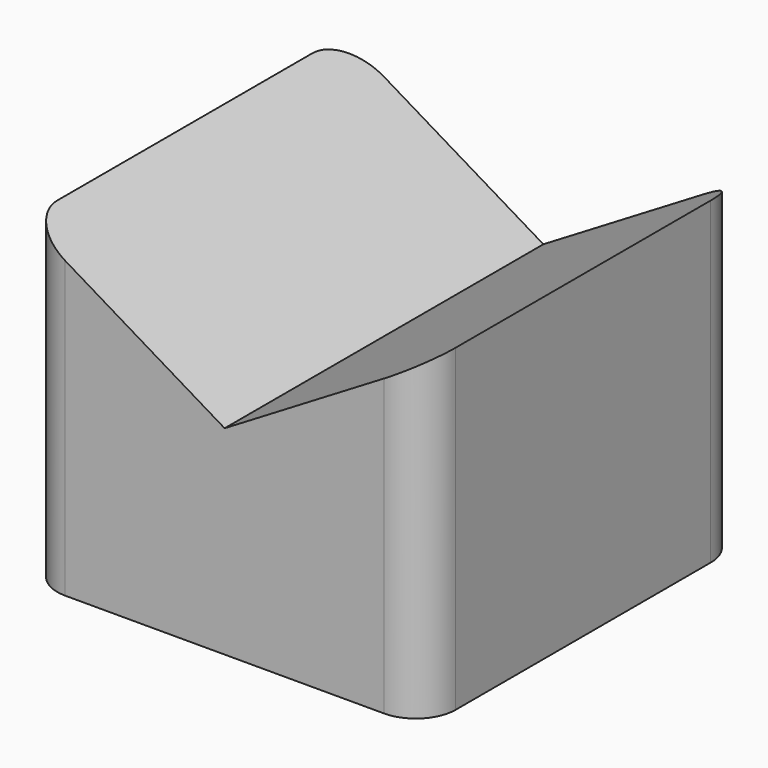
from build123d import *

# Parameters (mm, degrees)
F1_DEPTH = 20.32
F4_DEPTH = 25.4


with BuildPart() as f1:
    # F0 (on Top) → F1 (new body)
    with BuildSketch(Plane.XY):
        with BuildLine():
            Line((22.86, 0), (2.54, 0))
            ThreePointArc((2.54, 0), (0.7439487758, -0.7439487758), (0, -2.54))
            Line((0, -2.54), (0, -22.86))
            ThreePointArc((0, -22.86), (0.7439487758, -24.6560512242), (2.54, -25.4))
            Line((2.54, -25.4), (22.86, -25.4))
            ThreePointArc((22.86, -25.4), (24.6560512242, -24.6560512242), (25.4, -22.86))
            Line((25.4, -22.86), (25.4, -2.54))
            ThreePointArc((25.4, -2.54), (24.6560512242, -0.7439487758), (22.86, 0))
        make_face()
    extrude(amount=F1_DEPTH)

    # F2 (on face) → F4 (cut)
    with BuildSketch(Plane.XZ.offset(25.4)):
        Polygon((2.54, 18.796), (12.7, 12.7), (22.86, 18.796), (22.86, 20.32), (2.54, 20.32), align=None)
        Polygon((0, 20.32), (2.54, 18.796), (2.54, 20.32), align=None)
        Polygon((22.86, 20.32), (22.86, 18.796), (25.4, 20.32), align=None)
    extrude(amount=-F4_DEPTH, mode=Mode.SUBTRACT)


solid = f1.part
